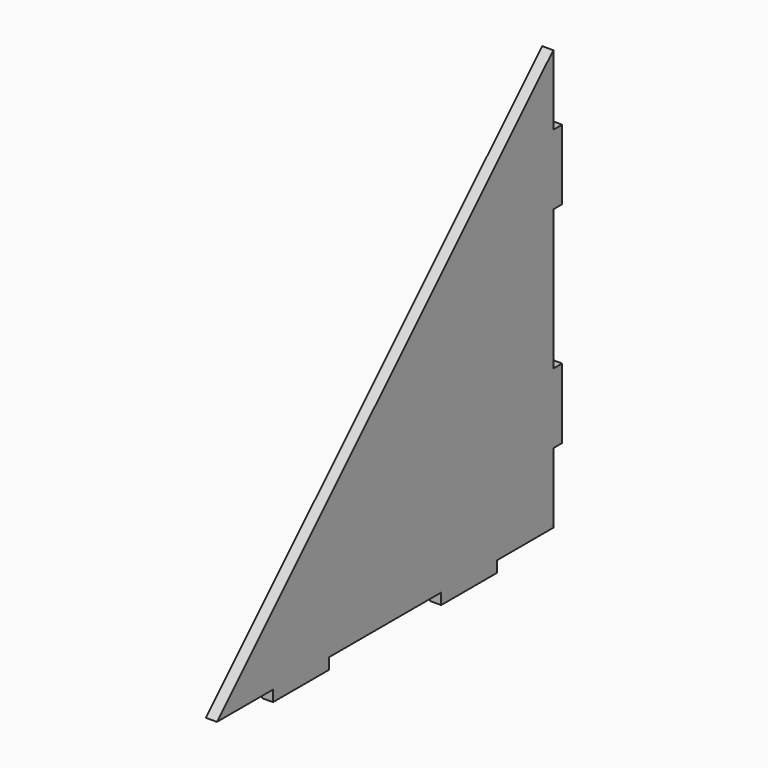
from build123d import *

# Parameters (mm, degrees)
F0_W     = 10
F0_H     = 1.5875
F0_W_2   = 1.5875
F0_H_2   = 10
F1_DEPTH = 1.5875


# Not quite as in the source:
# - a length typed as a fraction of an inch, garbled in the dataset ("3 / 203.2 mm" for 3/8 in), is restored


with BuildPart() as f1:
    # F0 (on Right) → F1 (new body)
    with BuildSketch(Plane.YZ):
        Polygon((15.5766666667, 44.4233333333), (-44.4233333333, -15.5766666667), (-34.4233333333, -15.5766666667), (-24.4233333333, -15.5766666667), (-4.4233333333, -15.5766666667), (5.5766666667, -15.5766666667), (15.5766666667, -15.5766666667), (15.5766666667, -5.5766666667), (15.5766666667, 4.4233333333), (15.5766666667, 24.4233333333), (15.5766666667, 34.4233333333), align=None)
        with Locations((-29.4233333333, -16.3704166667)):
            Rectangle(F0_W, F0_H)
        with Locations((16.3704166667, 29.4233333333)):
            Rectangle(F0_W_2, F0_H_2)
        with Locations((0.5766666667, -16.3704166667)):
            Rectangle(F0_W, F0_H)
        with Locations((16.3704166667, -0.5766666667)):
            Rectangle(F0_W_2, F0_H_2)
    extrude(amount=F1_DEPTH)


solid = f1.part
